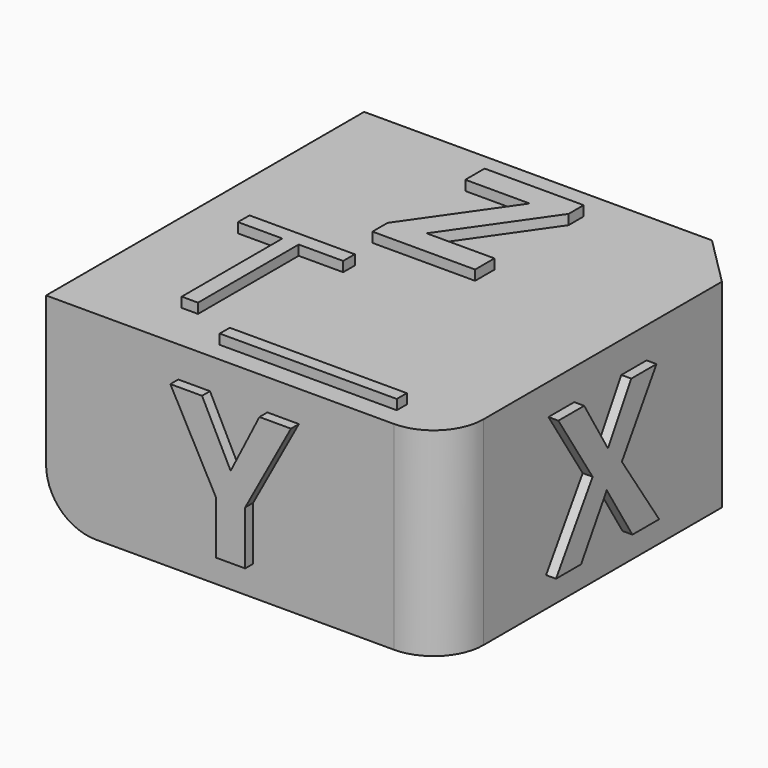
from build123d import *

# Parameters (mm, degrees)
F0_W          = 40
F0_H          = 40
F1_DEPTH      = 20
F2_R          = 5
F3_SIZE       = 5
F4_TEXT_SIZE  = 19.4444444444
F5_DEPTH      = 1
F6_TEXT_SIZE  = 19.4444444444
F7_DEPTH      = 1
F8_TEXT_SIZE  = 19.4444444444
F9_DEPTH      = 1
F10_R         = 5
F10_R_2       = 1.25
F10_R_3       = 2.5
F11_DEPTH     = 2
F10_W         = 8
F10_H         = 2
F10_TEXT_SIZE = 19.4444444444
F12_DEPTH     = 1
F13_TEXT_SIZE = 19.4444444444
F13_W         = 8.8677106944
F13_H         = 1.264166495
F13_W_2       = 0.0772717906
F14_DEPTH     = 1
F15_TEXT_SIZE = 36.1111111111
F16_DEPTH     = 1
F17_T1_DEPTH  = 65


# Not quite as in the source:
# - a fillet or chamfer that OpenCascade refuses, or shapes differently, is made with other operations: its cross-section is extruded or revolved along the edge and cut away or added
# - Text() gives the source's letters only with a copy of the font that has no kerning and outlines rounded to 1/6400 em; it was checked with that copy


with BuildPart() as f1:
    # F0 (on Top) → F1 (new body)
    with BuildSketch(Plane.XY):
        Rectangle(F0_W, F0_H)
    extrude(amount=F1_DEPTH)

    # F2
    f2_edges = [f1.edges().sort_by_distance(p)[0] for p in [
        (20, -20, 10),
    ]]
    fillet(f2_edges, radius=F2_R)

    # F3
    f3_edges = [f1.edges().sort_by_distance(p)[0] for p in [
        (20, 20, 10),
    ]]
    chamfer(f3_edges, length=F3_SIZE)

    # F4 (on face) → F5 (join)
    with BuildSketch(Plane.XZ.offset(20)):
        with Locations((-6.6976996528, 3)):
            Text('Y', F4_TEXT_SIZE, font='Open Sans', font_style=FontStyle.BOLD, text_align=(TextAlign.LEFT, TextAlign.BOTTOM))
    extrude(amount=F5_DEPTH)

    # F6 (on face) → F7 (cut)
    with BuildSketch(Plane(origin=(0, 20, 0), x_dir=(-1, 0, 0), z_dir=(0, 1, 0))):
        with Locations((-9.8255208333, 3)):
            Text('-Y', F6_TEXT_SIZE, font='Open Sans', font_style=FontStyle.BOLD, text_align=(TextAlign.LEFT, TextAlign.BOTTOM))
    extrude(amount=-F7_DEPTH, mode=Mode.SUBTRACT)

    # F8 (on face) → F9 (join)
    with BuildSketch(Plane.YZ.offset(20)):
        with Locations((-7.1154513889, 3)):
            Text('X', F8_TEXT_SIZE, font='Open Sans', font_style=FontStyle.BOLD, text_align=(TextAlign.LEFT, TextAlign.BOTTOM))
    extrude(amount=F9_DEPTH)

    # F10 (on face) → F11 (cut)
    with BuildSketch(Plane(origin=(-20, 0, 0), x_dir=(0, -1, 0), z_dir=(-1, 0, 0))):
        with Locations((-10, 10)):
            Circle(F10_R)
        with Locations((0, 3.75)):
            Circle(F10_R_2)
        with Locations((0, 15)):
            Circle(F10_R_3)
    extrude(amount=-F11_DEPTH, mode=Mode.SUBTRACT)

    # F10 (on face) → F12 (cut)
    with BuildSketch(Plane(origin=(-20, 0, 0), x_dir=(0, -1, 0), z_dir=(-1, 0, 0))):
        with Locations((0, 10)):
            Rectangle(F10_W, F10_H)
        with Locations((5.7690972222, 3)):
            Text('X', F10_TEXT_SIZE, font='Open Sans', font_style=FontStyle.BOLD, text_align=(TextAlign.LEFT, TextAlign.BOTTOM))
    extrude(amount=-F12_DEPTH, mode=Mode.SUBTRACT)

    # F13 (on face) → F14 (join)
    with BuildSketch(Plane.XY.offset(20)):
        with Locations((-6.0277777778, 3)):
            Text('Z', F13_TEXT_SIZE, font='Open Sans', font_style=FontStyle.BOLD, text_align=(TextAlign.LEFT, TextAlign.BOTTOM))
        Polygon((-10.3544199464, -15), (-8.7131671131, -15), (-8.7131671131, -2.3366989491), (-4.2406758706, -2.3366989491), (-4.2406758706, -0.8778075417), (-14.826911189, -0.8778075417), (-14.826911189, -2.3366989491), (-10.3544199464, -2.3366989491), align=None)
        with Locations((9.2834329281, -17.4093344323)):
            Rectangle(F13_W, F13_H)
        with Locations((0.338450443, -17.4093344323)):
            Rectangle(F13_W, F13_H)
        with Locations((4.8109416856, -17.4093344323)):
            Rectangle(F13_W_2, F13_H)
    extrude(amount=F14_DEPTH)

    # F15 (on face) → F16 (cut)
    with BuildSketch(Plane(origin=(0, 0, 0), x_dir=(1, 0, 0), z_dir=(0, 0, -1))):
        with Locations((-17.0510853237, -13)):
            Text('-Z', F15_TEXT_SIZE, font='Open Sans', font_style=FontStyle.BOLD, text_align=(TextAlign.LEFT, TextAlign.BOTTOM))
    extrude(amount=-F16_DEPTH, mode=Mode.SUBTRACT)

    # F17: fillet of radius 5 on 1 edges, made by hand

    # F17_s2 → F17_t1 (cut)
    with BuildSketch(Plane.XZ.offset(-32.5)):
        with BuildLine():
            ThreePointArc((-15, 0), (-18.5355339059, 1.4644660941), (-20, 5))
            Line((-20, 5), (-20, 0))
            Line((-20, 0), (-15, 0))
        make_face()
    extrude(amount=F17_T1_DEPTH, mode=Mode.SUBTRACT)


solid = f1.part
